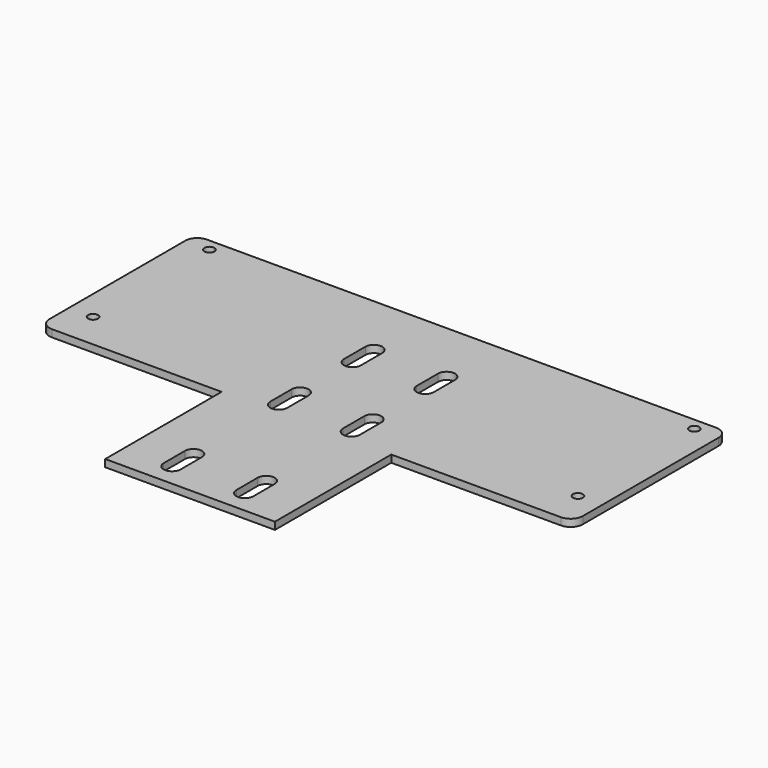
from build123d import *

# Parameters (mm, degrees)
F0_W     = 70
F0_H     = 60
F0_W_2   = 220
F0_H_2   = 50
F1_DEPTH = 3
F2_R     = 2.05
F3_DEPTH = 25
F4_R     = 5


# Not quite as in the source:
# - a feature names something its author has since deleted; it is built from what else it names


with BuildPart() as f1:
    # F0 (on Top) → F1 (new body)
    with BuildSketch(Plane.XY):
        Polygon((35, -15), (110, -15), (110, 15), (-110, 15), (-110, -15), (-35, -15), align=None)
        with Locations((0, -45)):
            Rectangle(F0_W, F0_H)
        with Locations((0, 40)):
            Rectangle(F0_W_2, F0_H_2)
    extrude(amount=F1_DEPTH)

    # F2 (on face) → F3 (cut)
    with BuildSketch(Plane.XY.offset(3)):
        with Locations((-100, 0)):
            Circle(F2_R)
        with Locations((100, 0)):
            Circle(F2_R)
        with BuildLine():
            ThreePointArc((-18.5, 27.5), (-15, 24), (-11.5, 27.5))
            Line((-11.5, 27.5), (-11.5, 38.5))
            ThreePointArc((-11.5, 38.5), (-15, 42), (-18.5, 38.5))
            Line((-18.5, 38.5), (-18.5, 27.5))
        make_face()
        with BuildLine():
            ThreePointArc((11.5, 27.5), (15, 24), (18.5, 27.5))
            Line((18.5, 27.5), (18.5, 38.5))
            ThreePointArc((18.5, 38.5), (15, 42), (11.5, 38.5))
            Line((11.5, 38.5), (11.5, 27.5))
        make_face()
        with BuildLine():
            ThreePointArc((-18.5, -65.5), (-15, -69), (-11.5, -65.5))
            Line((-11.5, -65.5), (-11.5, -54.5))
            ThreePointArc((-11.5, -54.5), (-15, -51), (-18.5, -54.5))
            Line((-18.5, -54.5), (-18.5, -65.5))
        make_face()
        with BuildLine():
            ThreePointArc((11.5, -65.5), (15, -69), (18.5, -65.5))
            Line((18.5, -65.5), (18.5, -54.5))
            ThreePointArc((18.5, -54.5), (15, -51), (11.5, -54.5))
            Line((11.5, -54.5), (11.5, -65.5))
        make_face()
        with Locations((-100, 60)):
            Circle(F2_R)
        with Locations((100, 60)):
            Circle(F2_R)
        with BuildLine():
            ThreePointArc((-18.5, -10.5), (-15, -14), (-11.5, -10.5))
            Line((-11.5, -10.5), (-11.5, 0.5))
            ThreePointArc((-11.5, 0.5), (-15, 4), (-18.5, 0.5))
            Line((-18.5, 0.5), (-18.5, -10.5))
        make_face()
        with BuildLine():
            ThreePointArc((11.5, -10.5), (15, -14), (18.5, -10.5))
            Line((18.5, -10.5), (18.5, 0.5))
            ThreePointArc((18.5, 0.5), (15, 4), (11.5, 0.5))
            Line((11.5, 0.5), (11.5, -10.5))
        make_face()
    extrude(amount=-F3_DEPTH, mode=Mode.SUBTRACT)

    # F4
    f4_edges = [f1.edges().sort_by_distance(p)[0] for p in [
        (-110, -15, 1.5),
        (110, -15, 1.5),
        (110, 65, 1.5),
        (-110, 65, 1.5),
    ]]
    fillet(f4_edges, radius=F4_R)


solid = f1.part
